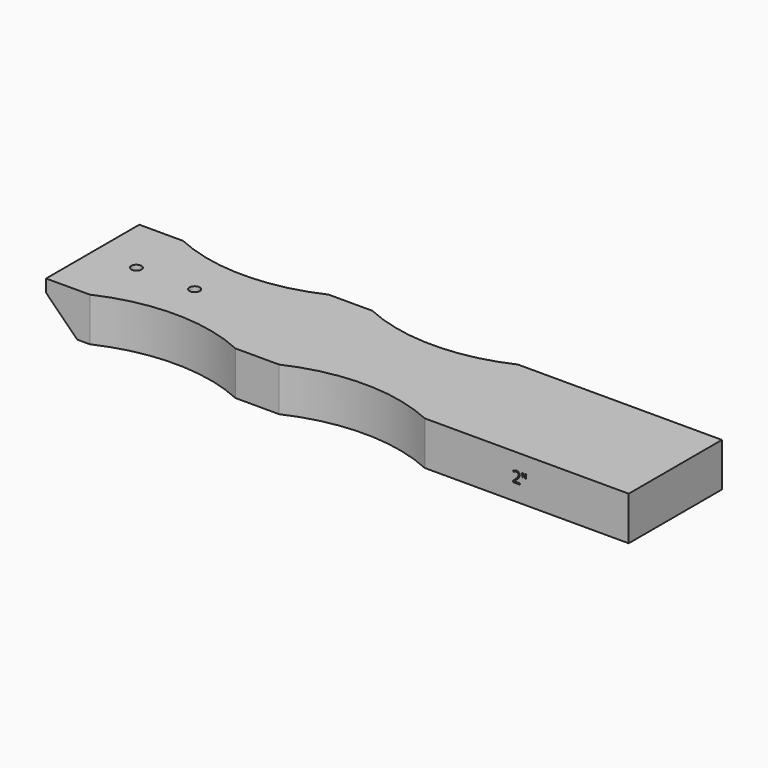
from build123d import *

# Parameters (mm, degrees)
F1_DEPTH     = 50.8
F3_D         = 4.445
F5_D         = 9.525
F5_DEPTH     = 5.08
F5_TIP       = 2.8615986981
F6_TEXT_SIZE = 6.7733333333
F7_DEPTH     = 2.54
F8_TEXT_SIZE = 6.7733333333
F9_DEPTH     = 2.54
F11_DEPTH    = 19.0510001


# Not quite as in the source:
# - Text() gives the source's letters only with a copy of the font that has no kerning and outlines rounded to 1/6400 em; it was checked with that copy


with BuildPart() as f1:
    # F0 (on Front) → F1 (new body)
    with BuildSketch(Plane.XZ):
        Polygon((124.8049397469, -23.8991970951), (-129.1950602531, -23.8991970951), (-129.1950602531, -29.3723903596), (-115.6182535177, -42.9491970951), (124.8049397469, -42.9491970951), align=None)
    extrude(amount=F1_DEPTH)

    # F3 (through all)
    with Locations(Plane.XY):
        with Locations((-110.1450602531, -25.4), (-84.7450602531, -25.4)):
            Hole(F3_D / 2)

    # F5
    with Locations(Plane(origin=(0, 0, -42.9491970951), x_dir=(1, 0, 0), z_dir=(0, 0, -1))):
        with Locations((-110.1450602531, 25.4), (-84.7450602531, 25.4)):
            Hole(F5_D / 2, depth=F5_DEPTH)
            with Locations((0, 0, -(F5_DEPTH + F5_TIP / 2))):  # 118° drill point
                Cone(0, F5_D / 2, F5_TIP, mode=Mode.SUBTRACT)

    # F6 (on face) → F7 (cut)
    with BuildSketch(Plane.XZ.offset(50.8)):
        with Locations((74.0049397469, -35.8625970951)):
            Text('2"', F6_TEXT_SIZE, font='Open Sans', text_align=(TextAlign.LEFT, TextAlign.BOTTOM))
    extrude(amount=-F7_DEPTH, mode=Mode.SUBTRACT)

    # F8 (on face) → F9 (cut)
    with BuildSketch(Plane(origin=(0, 0, 0), x_dir=(-1, 0, 0), z_dir=(0, 1, 0))):
        with Locations((-80.1527980802, -35.8625970951)):
            Text('2"', F8_TEXT_SIZE, font='Open Sans', text_align=(TextAlign.LEFT, TextAlign.BOTTOM))
    extrude(amount=-F9_DEPTH, mode=Mode.SUBTRACT)

    # F10 (on face) → F11 (cut, through all)
    with BuildSketch(Plane.XY.offset(-23.8991970951)):
        with BuildLine():
            Line((-46.6450602531, 0), (-110.1450602531, 0))
            ThreePointArc((-110.1450602531, 0), (-78.3950602531, -6.9296780721), (-46.6450602531, 0))
        make_face()
        with BuildLine():
            ThreePointArc((-27.5950602531, 0), (4.1549397469, -6.9296780721), (35.9049397469, 0))
            Line((35.9049397469, 0), (-27.5950602531, 0))
        make_face()
        with BuildLine():
            ThreePointArc((35.9049397469, -50.8), (4.1549397469, -43.8703219279), (-27.5950602531, -50.8))
            Line((-27.5950602531, -50.8), (35.9049397469, -50.8))
        make_face()
        with BuildLine():
            Line((-110.1450602531, -50.8), (-46.6450602531, -50.8))
            ThreePointArc((-46.6450602531, -50.8), (-78.3950602531, -43.8703219279), (-110.1450602531, -50.8))
        make_face()
    extrude(amount=-F11_DEPTH, mode=Mode.SUBTRACT)


solid = f1.part
